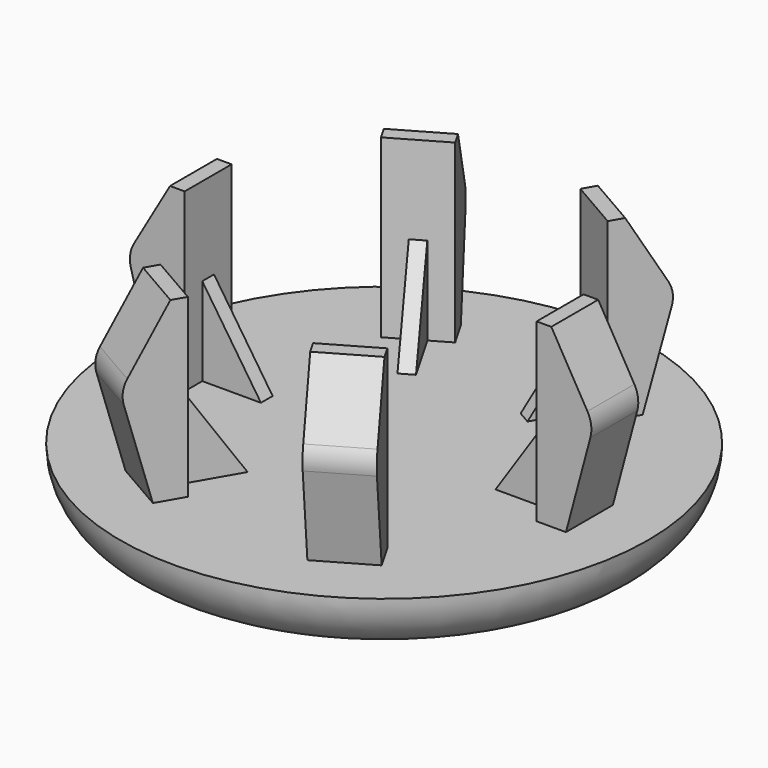
from build123d import *

# Parameters (mm, degrees)
F1_DEPTH        = 1
F1_COPIES_COUNT = 6
F2_DEPTH        = 0.25
F2_COPIES_COUNT = 6
F3_R            = 9
F4_DEPTH        = 2
F5_R            = 1.99999


# Not quite as in the source:
# - a fillet or chamfer is up to 0.001 mm smaller than in the source, because OpenCascade refuses the exact size
# - a pattern or mirror of a feature is missing from the dataset's text; its kind, count and spacing are read off the source's solid


with BuildPart() as f1:
    # F0 (on Front) → F1 (new body, symmetric)
    with BuildSketch(Plane.XZ):
        with BuildLine():
            Line((6, 3), (6, 0))
            Line((6, 0), (7, 0))
            Line((7, 0), (7.8323762036, 3.1064702829))
            ThreePointArc((7.8323762036, 3.1064702829), (7.8578952387, 3.4958155202), (7.7324757811, 3.865289328))
            Line((7.7324757811, 3.865289328), (6.5, 6))
            Line((6.5, 6), (6, 6))
            Line((6, 6), (6, 3))
        make_face()
    extrude(amount=F1_DEPTH, both=True)


with BuildPart() as f1_copies_1:
    # F1_copies: instance of F1
    add(f1.part.rotate(Axis((0, 0, 0), (0, 0, 1)), 1 * 360 / F1_COPIES_COUNT))


with BuildPart() as f1_copies_2:
    # F1_copies: instance of F1
    add(f1.part.rotate(Axis((0, 0, 0), (0, 0, 1)), 2 * 360 / F1_COPIES_COUNT))


with BuildPart() as f1_copies_3:
    # F1_copies: instance of F1
    add(f1.part.rotate(Axis((0, 0, 0), (0, 0, 1)), 3 * 360 / F1_COPIES_COUNT))


with BuildPart() as f1_copies_4:
    # F1_copies: instance of F1
    add(f1.part.rotate(Axis((0, 0, 0), (0, 0, 1)), 4 * 360 / F1_COPIES_COUNT))


with BuildPart() as f1_copies_5:
    # F1_copies: instance of F1
    add(f1.part.rotate(Axis((0, 0, 0), (0, 0, 1)), 5 * 360 / F1_COPIES_COUNT))


with BuildPart() as f1_1:
    add(f1.part)

    # F0 (on Front) → F2 (join, symmetric)
    with BuildSketch(Plane.XZ):
        Polygon((6, 3), (4, 0), (6, 0), align=None)
    f2 = extrude(amount=F2_DEPTH, both=True)

    # F2_copies: F2 ×6 about axis
    f2_copies_axis = Axis((0, 0, 0), (0, 0, 1))
    for i in range(1, F2_COPIES_COUNT):
        add(f2.rotate(f2_copies_axis, i * 360 / F2_COPIES_COUNT))

    add(f1_copies_1.part)  # F4 merges F1_copies_1

    add(f1_copies_2.part)  # F4 merges F1_copies_2

    add(f1_copies_3.part)  # F4 merges F1_copies_3

    add(f1_copies_4.part)  # F4 merges F1_copies_4

    add(f1_copies_5.part)  # F4 merges F1_copies_5
    # F3 (on Top) → F4 (join)
    with BuildSketch(Plane.XY):
        Circle(F3_R)
    extrude(amount=-F4_DEPTH)

    # F5 (radius 2 in the source; OpenCascade refuses exactly that, so slightly less here)
    f5_edges = [f1_1.edges().sort_by_distance(p)[0] for p in [
        (-9, 0, -2),
    ]]
    fillet(f5_edges, radius=F5_R)


solid = f1_1.part
